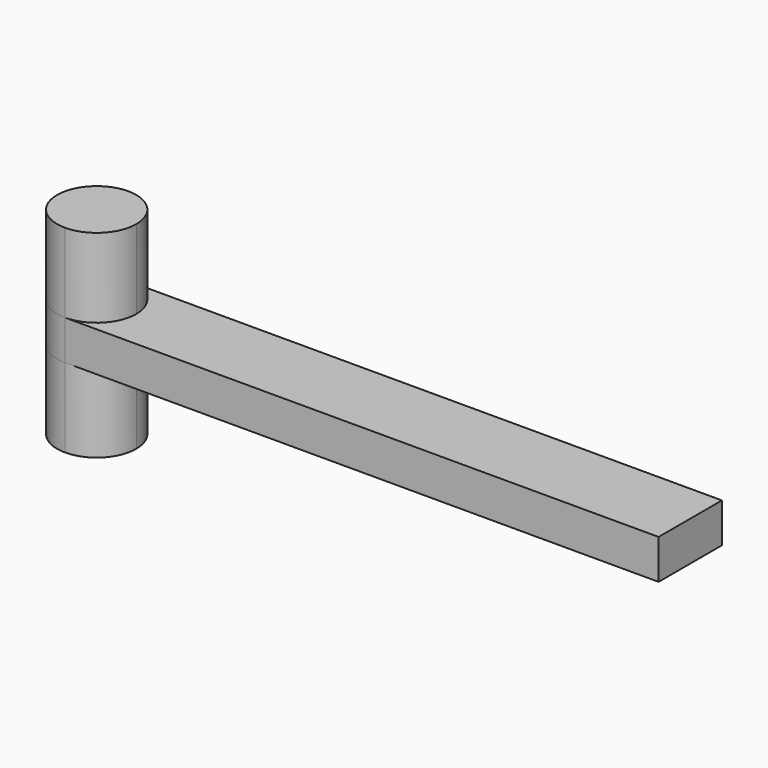
from build123d import *

# Parameters (mm, degrees)
F0_W     = 23.1644526571
F0_H     = 12.7
F0_W_2   = 78.4355473429
F1_DEPTH = 6.35
F3_DEPTH = 12.7
F5_DEPTH = 12.7
F6_R     = 6.35
F7_R     = 6.3499
F8_R     = 6.35
F9_DEPTH = 25.4


# Not quite as in the source:
# - a fillet or chamfer is up to 0.001 mm smaller than in the source, because OpenCascade refuses the exact size


with BuildPart() as f1:
    # F0 (on Top) → F1 (new body)
    with BuildSketch(Plane.XY):
        with Locations((-39.2177736714, 0)):
            Rectangle(F0_W, F0_H)
        with Locations((11.5822263286, 0)):
            Rectangle(F0_W_2, F0_H)
    extrude(amount=F1_DEPTH)

    # F2 (on face) → F3 (join)
    with BuildSketch(Plane(origin=(0, 0, 0), x_dir=(1, 0, 0), z_dir=(0, 0, -1))):
        with BuildLine():
            ThreePointArc((-44.45, -6.35), (-39.9598719395, -4.4901280605), (-38.1, 0))
            ThreePointArc((-38.1, 0), (-39.9598719395, 4.4901280605), (-44.45, 6.35))
            ThreePointArc((-44.45, 6.35), (-48.9401280605, 4.4901280605), (-50.8, 0))
            ThreePointArc((-50.8, 0), (-48.9401280605, -4.4901280605), (-44.45, -6.35))
        make_face()
    extrude(amount=F3_DEPTH)

    # F4 (on face) → F5 (join)
    with BuildSketch(Plane.XY.offset(6.35)):
        with BuildLine():
            ThreePointArc((-44.45, -6.35), (-39.9598719395, -4.4901280605), (-38.1, 0))
            ThreePointArc((-38.1, 0), (-39.9598719395, 4.4901280605), (-44.45, 6.35))
            ThreePointArc((-44.45, 6.35), (-48.9401280605, 4.4901280605), (-50.8, 0))
            ThreePointArc((-50.8, 0), (-48.9401280605, -4.4901280605), (-44.45, -6.35))
        make_face()
    extrude(amount=F5_DEPTH)

    # F6
    f6_edges = [f1.edges().sort_by_distance(p)[0] for p in [
        (-50.8, 6.35, 3.175),
    ]]
    fillet(f6_edges, radius=F6_R)

    # F7 (radius 6.35 in the source; OpenCascade refuses exactly that, so slightly less here)
    f7_edges = [f1.edges().sort_by_distance(p)[0] for p in [
        (-50.8, -6.35, 3.175),
    ]]
    fillet(f7_edges, radius=F7_R)

    # F8 (on face) → F9 (cut)
    with BuildSketch(Plane.XY.offset(6.35)):
        with Locations((63.4561311297, 1.0546775941)):
            Circle(F8_R)
    extrude(amount=-F9_DEPTH, mode=Mode.SUBTRACT)


solid = f1.part
